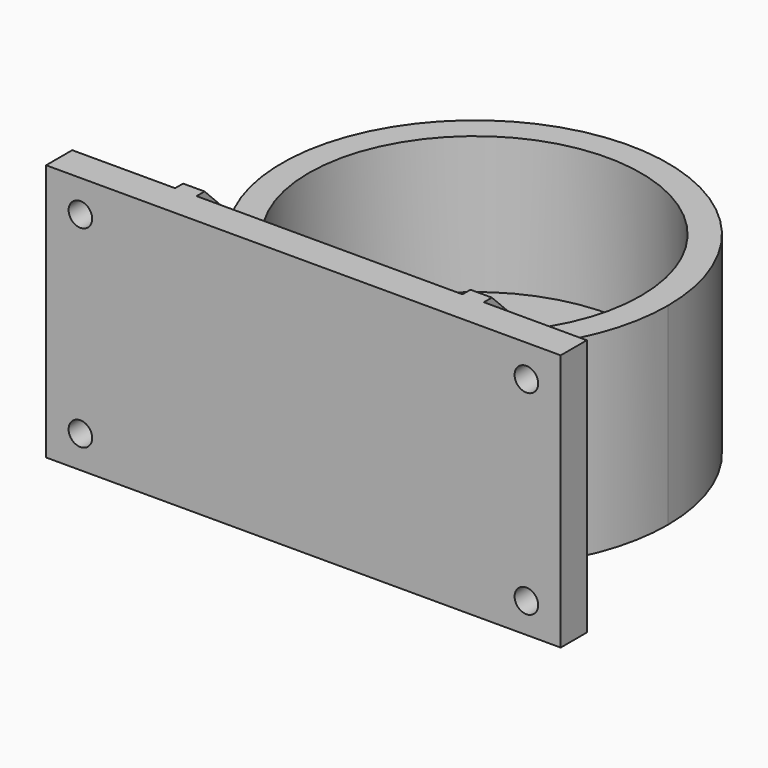
from build123d import *

# Parameters (mm, degrees)
F0_W      = 24
F0_H      = 7.6146386564
F1_DEPTH  = 45
F2_R      = 38.75
F4_DEPTH  = 32
F5_DEPTH  = 15
F7_DEPTH  = 15
F8_SIZE   = 14.99999
F9_R      = 2.75
F10_DEPTH = 25
F11_R     = 22.5
F12_DEPTH = 25


# Not quite as in the source:
# - a fillet or chamfer is up to 0.001 mm smaller than in the source, because OpenCascade refuses the exact size


with BuildPart() as f1:
    # F0 (on Top) → F1 (new body)
    with BuildSketch(Plane.XY):
        with BuildLine():
            ThreePointArc((36, -27), (42.6907484123, -14.2302494708), (45, 0))
            ThreePointArc((45, 0), (-14.2302494708, 42.6907484123), (-36, -27))
            Line((-36, -27), (36, -27))
        make_face()
        with BuildLine():
            ThreePointArc((-15.1652218257, -42.3676297069), (-26.7116265289, -36.2144861648), (-36, -27))
            Line((-36, -27), (-36, -42.3676297069))
            Line((-36, -42.3676297069), (-15.1652218257, -42.3676297069))
        make_face()
        with BuildLine():
            Line((36, -27), (-36, -27))
            ThreePointArc((-36, -27), (-26.7116265289, -36.2144861648), (-15.1652218257, -42.3676297069))
            Line((-15.1652218257, -42.3676297069), (15.1652218257, -42.3676297069))
            ThreePointArc((15.1652218257, -42.3676297069), (26.7116265289, -36.2144861648), (36, -27))
        make_face()
        with BuildLine():
            Line((15.1652218257, -42.3676297069), (-15.1652218257, -42.3676297069))
            ThreePointArc((-15.1652218257, -42.3676297069), (0, -45), (15.1652218257, -42.3676297069))
        make_face()
        with Locations((-48, -46.174949035)):
            Rectangle(F0_W, F0_H)
        with BuildLine():
            ThreePointArc((15.1652218257, -42.3676297069), (0, -45), (-15.1652218257, -42.3676297069))
            Line((-15.1652218257, -42.3676297069), (-36, -42.3676297069))
            Line((-36, -42.3676297069), (-36, -49.9822683632))
            Line((-36, -49.9822683632), (36, -49.9822683632))
            Line((36, -49.9822683632), (36, -42.3676297069))
            Line((36, -42.3676297069), (15.1652218257, -42.3676297069))
        make_face()
        with Locations((48, -46.174949035)):
            Rectangle(F0_W, F0_H)
        with BuildLine():
            Line((36, -42.3676297069), (36, -27))
            ThreePointArc((36, -27), (26.7116265289, -36.2144861648), (15.1652218257, -42.3676297069))
            Line((15.1652218257, -42.3676297069), (36, -42.3676297069))
        make_face()
    extrude(amount=F1_DEPTH)

    # F2 (on face) → F4 (cut)
    with BuildSketch(Plane.XY.offset(45)):
        Circle(F2_R)
    extrude(amount=-F4_DEPTH, mode=Mode.SUBTRACT)

    # F3 (on face) → F5 (join)
    with BuildSketch(Plane.XY.offset(45)):
        Polygon((-36, -42.3676297069), (-60, -42.3676297069), (-60, -49.9822683632), (60, -49.9822683632), (60, -42.3676297069), (36, -42.3676297069), align=None)
    extrude(amount=F5_DEPTH)

    # F6 (on face) → F7 (join)
    with BuildSketch(Plane.XY.offset(45)):
        Polygon((-31, -25.031657964), (-36, -25.031657964), (-36, -27), (-36, -42.3676297069), (-31, -42.3676297069), align=None)
        Polygon((36, -42.3676297069), (36, -27), (36, -25.031657964), (31, -25.031657964), (31, -42.3676297069), align=None)
    extrude(amount=F7_DEPTH)

    # F8 (size 15 in the source; OpenCascade refuses exactly that, so slightly less here)
    f8_edges = [f1.edges().sort_by_distance(p)[0] for p in [
        (-33.5, -25.031658, 60),
        (33.5, -25.031658, 60),
    ]]
    chamfer(f8_edges, length=F8_SIZE)

    # F9 (on face) → F10 (cut)
    with BuildSketch(Plane(origin=(0, -42.3676297069, 0), x_dir=(-1, 0, 0), z_dir=(0, 1, 0))):
        with Locations((52, 7.5)):
            Circle(F9_R)
        with Locations((52, 52.5)):
            Circle(F9_R)
        with Locations((-52, 7)):
            Circle(F9_R)
        with Locations((-52, 52.5)):
            Circle(F9_R)
    extrude(amount=-F10_DEPTH, mode=Mode.SUBTRACT)

    # F11 (on face) → F12 (cut)
    with BuildSketch(Plane.XY.offset(13)):
        Circle(F11_R)
    extrude(amount=-F12_DEPTH, mode=Mode.SUBTRACT)


solid = f1.part
